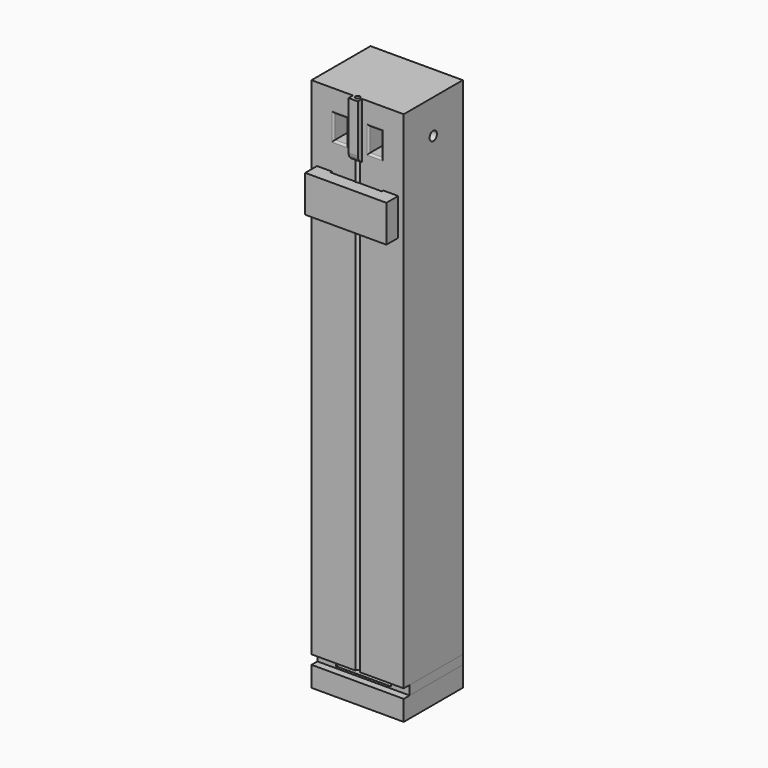
from build123d import *

# Parameters (mm, degrees)
F0_W         = 127
F0_H         = 27.94
F1_DEPTH     = 101.6
F0_W_2       = 20.32
F0_H_2       = 50.8
F0_W_3       = 57.15
F0_H_3       = 76.2
F0_W_4       = 17.78
F0_H_4       = 33.02
F3_R         = 2.54
F0_H_5       = 12.7
F0_W_5       = 76.2
F0_H_6       = 8.89
F4_DEPTH     = 91.44
F6_D         = 12.7
F6_DEPTH     = 693.42
F6_TIP       = 3.8154649308
F0_W_6       = 12.7
F7_DEPTH     = 109.22
F8_T1_DEPTH  = 61.8868884968
F9_DEPTH     = 121.92
F10_W        = 17.78
F10_H        = 50.8
F11_DEPTH    = 71.12
F12_D        = 6.35
F12_DEPTH    = 701.04
F12_TIP      = 1.9077324654
F13_T1_DEPTH = 59.055
F13_T3_DEPTH = 59.055


# Not quite as in the source:
# - a fillet or chamfer that OpenCascade refuses, or shapes differently, is made with other operations: its cross-section is extruded or revolved along the edge and cut away or added
# - a feature names something its author has since deleted; it is built from what else it names


with BuildPart() as f1:
    # F0 (on Front) → F1 (new body)
    with BuildSketch(Plane.XZ):
        with Locations((-20.794781892, -69.4378848389)):
            Rectangle(F0_W, F0_H)
    extrude(amount=F1_DEPTH)


with BuildPart() as f1b:
    # F0 (on Front) → F1, piece 2 (new body)
    with BuildSketch(Plane.XZ):
        Polygon((-27.144781892, 576.9921151611), (-84.294781892, 576.9921151611), (-84.294781892, -42.7678848389), (42.705218108, -42.7678848389), (42.705218108, 576.9921151611), (-14.444781892, 576.9921151611), align=None)
        with Locations((-66.514781892, 526.1921151611)):
            Rectangle(F0_W_2, F0_H_2, mode=Mode.SUBTRACT)
        with Locations((24.925218108, 526.1921151611)):
            Rectangle(F0_W_2, F0_H_2, mode=Mode.SUBTRACT)
        with Locations((14.130218108, 615.0921151611)):
            Rectangle(F0_W_3, F0_H_3)
        with Locations((3.335218108, 606.2021151611)):
            Rectangle(F0_W_4, F0_H_4, mode=Mode.SUBTRACT)
        with Locations((-55.719781892, 615.0921151611)):
            Rectangle(F0_W_3, F0_H_3)
        with Locations((-44.924781892, 606.2021151611)):
            Rectangle(F0_W_4, F0_H_4, mode=Mode.SUBTRACT)
    extrude(amount=F1_DEPTH)

    # F3
    f3_edges = [f1b.edges().sort_by_distance(p)[0] for p in [
        (12.225218, -101.6, 606.202115),
        (3.335218, -101.6, 589.692115),
        (-5.554782, -101.6, 606.202115),
        (3.335218, -101.6, 622.712115),
        (-36.034782, -101.6, 606.202115),
        (-44.924782, -101.6, 622.712115),
        (-53.814782, -101.6, 606.202115),
        (-44.924782, -101.6, 589.692115),
    ]]
    fillet(f3_edges, radius=F3_R)

    # F6
    with Locations(Plane(origin=(-84.294781892, 0, 0), x_dir=(0, -1, 0), z_dir=(-1, 0, 0))):
        with Locations((50.8, 606.2021151611)):
            Hole(F6_D / 2, depth=F6_DEPTH)
            with Locations((0, 0, -(F6_DEPTH + F6_TIP / 2))):  # 118° drill point
                Cone(0, F6_D / 2, F6_TIP, mode=Mode.SUBTRACT)

    # F0 (on Front) → F7 (join)
    with BuildSketch(Plane.XZ):
        with Locations((-20.794781892, 615.0921151611)):
            Rectangle(F0_W_6, F0_H_3)
    extrude(amount=F7_DEPTH)

    # F8: fillet of radius 10.16 on 1 edges, made by hand

    # F8_s2 → F8_t1 (cut)
    with BuildSketch(Plane.YZ.offset(-51.7382261404)):
        with BuildLine():
            ThreePointArc((-101.6, 576.9921151611), (-107.0921852568, 580.6077889138), (-109.22, 586.8294928604))
            Line((-109.22, 586.8294928604), (-109.22, 576.9921151611))
            Line((-109.22, 576.9921151611), (-101.6, 576.9921151611))
        make_face()
    extrude(amount=F8_T1_DEPTH, mode=Mode.SUBTRACT)

    # F0 (on Front) → F9 (join)
    with BuildSketch(Plane.XZ):
        with Locations((24.925218108, 526.1921151611)):
            Rectangle(F0_W_2, F0_H_2)
        with Locations((-66.514781892, 526.1921151611)):
            Rectangle(F0_W_2, F0_H_2)
    extrude(amount=F9_DEPTH)

    # F10 (on face) → F11 (join)
    with BuildSketch(Plane(origin=(14.765218108, 0, 0), x_dir=(0, -1, 0), z_dir=(-1, 0, 0))):
        with Locations((113.03, 526.1921151611)):
            Rectangle(F10_W, F10_H)
    extrude(amount=F11_DEPTH)

    # F12
    with Locations(Plane.XY.offset(653.1921151611)):
        with Locations((-20.794781892, -101.6)):
            Hole(F12_D / 2, depth=F12_DEPTH)
            with Locations((0, 0, -(F12_DEPTH + F12_TIP / 2))):  # 118° drill point
                Cone(0, F12_D / 2, F12_TIP, mode=Mode.SUBTRACT)

    # F13: fillet of radius 10.16 on 2 edges, made by hand

    # F13_s2 → F13_t1 (cut)
    with BuildSketch(Plane.YZ.offset(-56.354781892)):
        with BuildLine():
            ThreePointArc((-114.3, 500.7921151611), (-107.1157951031, 503.7679102642), (-104.14, 510.9521151611))
            Line((-104.14, 510.9521151611), (-104.14, 500.7921151611))
            Line((-104.14, 500.7921151611), (-114.3, 500.7921151611))
        make_face()
    extrude(amount=F13_T1_DEPTH, mode=Mode.SUBTRACT)

    # F13_s4 → F13_t3 (cut)
    with BuildSketch(Plane.YZ.offset(-44.289781892)):
        with BuildLine():
            ThreePointArc((-114.3, 500.7921151611), (-107.1157951031, 503.7679102642), (-104.14, 510.9521151611))
            Line((-104.14, 510.9521151611), (-104.14, 500.7921151611))
            Line((-104.14, 500.7921151611), (-114.3, 500.7921151611))
        make_face()
    extrude(amount=F13_T3_DEPTH, mode=Mode.SUBTRACT)


with BuildPart() as f4:
    # F0 (on Front) → F4 (new body)
    with BuildSketch(Plane.XZ):
        with Locations((-20.794781892, -49.1178848389)):
            Rectangle(F0_W, F0_H_5)
        with Locations((-20.794781892, -48.4828848389)):
            Rectangle(F0_W_5, F0_H_6, mode=Mode.SUBTRACT)
    extrude(amount=F4_DEPTH)


solid = Compound([f1.part, f1b.part, f4.part])
